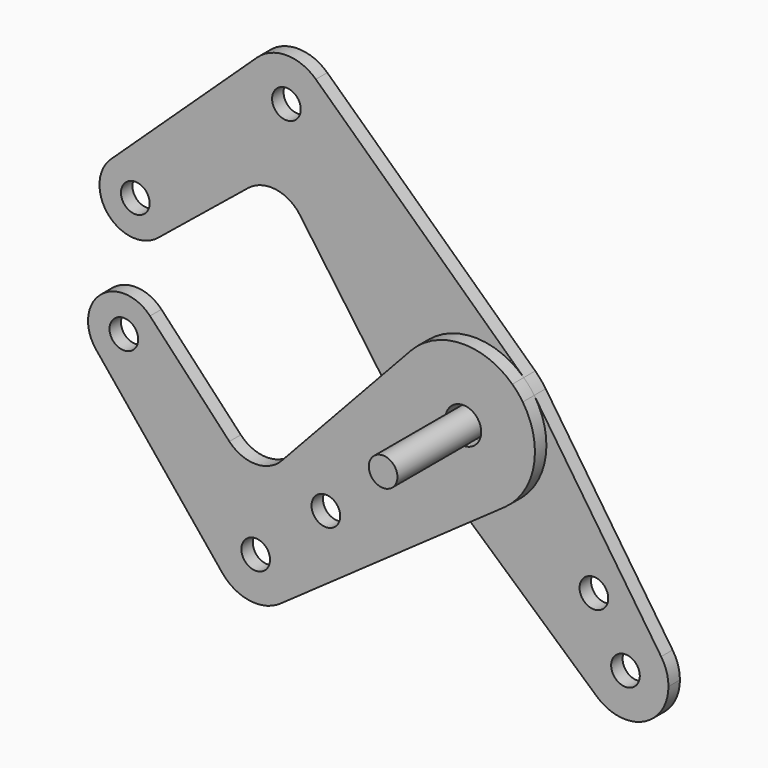
from build123d import *

# Parameters (mm, degrees)
F0_R     = 3.175
F0_R_2   = 3.96875
F1_DEPTH = 3.175
F2_DEPTH = 3.175
F3_DEPTH = 25.4


# Not quite as in the source:
# - a feature names something its author has since deleted; it is built from what else it names


with BuildPart() as f1:
    # F0 (on Front) → F1 (new body)
    with BuildSketch(Plane.XZ):
        with BuildLine():
            ThreePointArc((21.168407994, 17.4724150988), (32.2496948497, 22.5266363925), (43.6506851161, 18.2420719796))
            Line((43.6506851161, 18.2420719796), (-2.4416753004, 61.4557481855))
            ThreePointArc((-2.4416753004, 61.4557481855), (-0.2162960867, 58.2934233078), (0.5686178911, 54.5070634035))
            ThreePointArc((0.5686178911, 54.5070634035), (-12.7427420132, 45.7669773813), (-15.4710889174, 61.4557481855))
            Line((-15.4710889174, 61.4557481855), (-47.8775973584, 31.0731782742))
            ThreePointArc((-47.8775973584, 31.0731782742), (-39.2933750978, 32.5660126411), (-34.511175018, 25.2826076226))
            ThreePointArc((-34.511175018, 25.2826076226), (-35.2826057932, 21.8691990453), (-37.4469502912, 19.1192760553))
            Line((-37.4469502912, 19.1192760553), (-17.4168982381, 35.3742520435))
            ThreePointArc((-17.4168982381, 35.3742520435), (-11.3398687202, 37.0752466303), (-5.9425206073, 33.8053378098))
            Line((-5.9425206073, 33.8053378098), (12.3676167081, 8.0098658563))
            Line((12.3676167081, 8.0098658563), (21.168407994, 17.4724150988))
        make_face()
        with BuildLine():
            ThreePointArc((0.5686178911, 54.5070634035), (-0.2162960867, 58.2934233078), (-2.4416753004, 61.4557481855))
            ThreePointArc((-2.4416753004, 61.4557481855), (-8.9563821089, 64.0320634035), (-15.4710889174, 61.4557481855))
            ThreePointArc((-15.4710889174, 61.4557481855), (-12.7427420132, 45.7669773813), (0.5686178911, 54.5070634035))
        make_face()
        with Locations((-8.9563821089, 54.5070634035)):
            Circle(F0_R, mode=Mode.SUBTRACT)
        with BuildLine():
            ThreePointArc((-34.511175018, 25.2826076226), (-39.2933750978, 32.5660126411), (-47.8775973584, 31.0731782742))
            ThreePointArc((-47.8775973584, 31.0731782742), (-48.4294416089, 20.0639548045), (-37.4469502912, 19.1192760553))
            ThreePointArc((-37.4469502912, 19.1192760553), (-35.2826057932, 21.8691990453), (-34.511175018, 25.2826076226))
        make_face()
        with Locations((-42.448675018, 25.2826076226)):
            Circle(F0_R, mode=Mode.SUBTRACT)
        with BuildLine():
            ThreePointArc((48.6678404353, 6.6609306763), (47.9771603326, 11.292566916), (45.9652194266, 15.52118218))
            ThreePointArc((45.9652194266, 15.52118218), (44.8847270854, 16.9469358407), (43.6506851161, 18.2420719796))
            ThreePointArc((43.6506851161, 18.2420719796), (32.2496948497, 22.5266363925), (21.168407994, 17.4724150988))
            ThreePointArc((21.168407994, 17.4724150988), (16.9523480083, 7.7070782137), (19.8475346273, -2.5279039906))
            ThreePointArc((19.8475346273, -2.5279039906), (20.9635537477, -3.926023629), (22.229787853, -5.1897041229))
            ThreePointArc((22.229787853, -5.1897041229), (31.8827140076, -9.1879587134), (41.9298775136, -6.3209866871))
            ThreePointArc((41.9298775136, -6.3209866871), (46.8830158887, -0.6522478865), (48.6678404353, 6.6609306763))
        make_face()
        with Locations((32.7928404353, 6.6609306763)):
            Circle(F0_R_2, mode=Mode.SUBTRACT)
        with BuildLine():
            ThreePointArc((59.8543869213, -38.726356385), (59.9298350891, -24.4390555964), (74.0956458655, -26.2998246032))
            Line((74.0956458655, -26.2998246032), (45.9652194266, 15.52118218))
            ThreePointArc((45.9652194266, 15.52118218), (47.9771603326, 11.292566916), (48.6678404353, 6.6609306763))
            ThreePointArc((48.6678404353, 6.6609306763), (46.8830158887, -0.6522478865), (41.9298775136, -6.3209866871))
            Line((41.9298775136, -6.3209866871), (31.63109975, -13.5695549573))
            Line((31.63109975, -13.5695549573), (59.8543869213, -38.726356385))
        make_face()
        with Locations((59.1909500346, -18.7631345147)):
            Circle(F0_R, mode=Mode.SUBTRACT)
        with BuildLine():
            Line((22.229787853, -5.1897041229), (31.63109975, -13.5695549573))
            Line((31.63109975, -13.5695549573), (41.9298775136, -6.3209866871))
            ThreePointArc((41.9298775136, -6.3209866871), (31.8827140076, -9.1879587134), (22.229787853, -5.1897041229))
        make_face()
        with BuildLine():
            ThreePointArc((19.8475346273, -2.5279039906), (16.9523480083, 7.7070782137), (21.168407994, 17.4724150988))
            Line((21.168407994, 17.4724150988), (12.3676167081, 8.0098658563))
            Line((12.3676167081, 8.0098658563), (19.8475346273, -2.5279039906))
        make_face()
        with BuildLine():
            ThreePointArc((59.8543869213, -38.726356385), (70.088227935, -40.3077379996), (75.7172184707, -31.6159755055))
            ThreePointArc((75.7172184707, -31.6159755055), (75.3028104091, -28.8369937617), (74.0956458655, -26.2998246032))
            ThreePointArc((74.0956458655, -26.2998246032), (59.9298350891, -24.4390555964), (59.8543869213, -38.726356385))
        make_face()
        with Locations((66.1922184707, -31.6159755055)):
            Circle(F0_R, mode=Mode.SUBTRACT)
    extrude(amount=-F1_DEPTH)


with BuildPart() as f2:
    # F0 (on Front) → F2 (new body)
    with BuildSketch(Plane.XZ):
        with Locations((32.7928404353, 6.6609306763)):
            Circle(F0_R)
    extrude(amount=F2_DEPTH)

    # F0 (on Front) → F3 (join)
    with BuildSketch(Plane.XZ):
        with Locations((32.7928404353, 6.6609306763)):
            Circle(F0_R)
    extrude(amount=F3_DEPTH)


with BuildPart() as f2b:
    # F0 (on Front) → F2, piece 2 (new body)
    with BuildSketch(Plane.XZ):
        with BuildLine():
            ThreePointArc((48.6678404353, 6.6609306763), (47.9771603326, 11.292566916), (45.9652194266, 15.52118218))
            ThreePointArc((45.9652194266, 15.52118218), (44.8847270854, 16.9469358407), (43.6506851161, 18.2420719796))
            ThreePointArc((43.6506851161, 18.2420719796), (32.2496948497, 22.5266363925), (21.168407994, 17.4724150988))
            ThreePointArc((21.168407994, 17.4724150988), (16.9523480083, 7.7070782137), (19.8475346273, -2.5279039906))
            ThreePointArc((19.8475346273, -2.5279039906), (20.9635537477, -3.926023629), (22.229787853, -5.1897041229))
            ThreePointArc((22.229787853, -5.1897041229), (31.8827140076, -9.1879587134), (41.9298775136, -6.3209866871))
            ThreePointArc((41.9298775136, -6.3209866871), (46.8830158887, -0.6522478865), (48.6678404353, 6.6609306763))
        make_face()
        with Locations((32.7928404353, 6.6609306763)):
            Circle(F0_R_2, mode=Mode.SUBTRACT)
        with BuildLine():
            Line((-7.7419969901, -41.2814433271), (31.63109975, -13.5695549573))
            Line((31.63109975, -13.5695549573), (22.229787853, -5.1897041229))
            ThreePointArc((22.229787853, -5.1897041229), (20.9635537477, -3.926023629), (19.8475346273, -2.5279039906))
            Line((19.8475346273, -2.5279039906), (12.3676167081, 8.0098658563))
            Line((12.3676167081, 8.0098658563), (-7.4631189723, -13.3120024615))
            ThreePointArc((-7.4631189723, -13.3120024615), (-13.2594776313, -15.8437444101), (-19.0659058445, -13.3351825907))
            Line((-19.0659058445, -13.3351825907), (-36.6581043663, 5.4289223404))
            ThreePointArc((-36.6581043663, 5.4289223404), (-35.067395969, 2.9190111085), (-34.511175018, 0))
            ThreePointArc((-34.511175018, 0), (-39.7951432267, -7.4808204953), (-48.6120065852, -5.0017247268))
            Line((-48.6120065852, -5.0017247268), (-20.6202171177, -39.4943625812))
            ThreePointArc((-20.6202171177, -39.4943625812), (-20.0372197924, -26.8358187348), (-7.3956423811, -25.9588131796))
            ThreePointArc((-7.3956423811, -25.9588131796), (-4.6731134737, -29.2965551642), (-3.699219237, -33.4922929091))
            ThreePointArc((-3.699219237, -33.4922929091), (-4.3961637904, -37.0687523357), (-6.3850065401, -40.1218324621))
            ThreePointArc((-6.3850065401, -40.1218324621), (-7.0362782136, -40.7334952188), (-7.7419969901, -41.2814433271))
        make_face()
        with Locations((2.3257738993, -19.9237955822)):
            Circle(F0_R, mode=Mode.SUBTRACT)
        with BuildLine():
            Line((22.229787853, -5.1897041229), (31.63109975, -13.5695549573))
            Line((31.63109975, -13.5695549573), (41.9298775136, -6.3209866871))
            ThreePointArc((41.9298775136, -6.3209866871), (31.8827140076, -9.1879587134), (22.229787853, -5.1897041229))
        make_face()
        with BuildLine():
            ThreePointArc((-20.6202171177, -39.4943625812), (-14.533436061, -42.9268875643), (-7.7419969901, -41.2814433271))
            ThreePointArc((-7.7419969901, -41.2814433271), (-7.0362782136, -40.7334952188), (-6.3850065401, -40.1218324621))
            Line((-6.3850065401, -40.1218324621), (-6.8903244606, -33.0403228209))
            Line((-6.8903244606, -33.0403228209), (-7.3956423811, -25.9588131796))
            ThreePointArc((-7.3956423811, -25.9588131796), (-20.0372197924, -26.8358187348), (-20.6202171177, -39.4943625812))
        make_face()
        with BuildLine():
            ThreePointArc((-10.049219237, -33.4922929091), (-16.3972054455, -33.6053571438), (-10.0572718488, -33.266307865))
            ThreePointArc((-10.0572718488, -33.266307865), (-10.0512330286, -33.3792286743), (-10.049219237, -33.4922929091))
        make_face(mode=Mode.SUBTRACT)
        with BuildLine():
            ThreePointArc((19.8475346273, -2.5279039906), (16.9523480083, 7.7070782137), (21.168407994, 17.4724150988))
            Line((21.168407994, 17.4724150988), (12.3676167081, 8.0098658563))
            Line((12.3676167081, 8.0098658563), (19.8475346273, -2.5279039906))
        make_face()
        with BuildLine():
            Line((-6.8903244606, -33.0403228209), (-6.3850065401, -40.1218324621))
            ThreePointArc((-6.3850065401, -40.1218324621), (-4.3961637904, -37.0687523357), (-3.699219237, -33.4922929091))
            ThreePointArc((-3.699219237, -33.4922929091), (-4.6731134737, -29.2965551642), (-7.3956423811, -25.9588131796))
            Line((-7.3956423811, -25.9588131796), (-6.8903244606, -33.0403228209))
        make_face()
        with BuildLine():
            ThreePointArc((-36.6581043663, 5.4289223404), (-47.667327836, 5.9807665909), (-48.6120065852, -5.0017247268))
            ThreePointArc((-48.6120065852, -5.0017247268), (-39.7951432267, -7.4808204953), (-34.511175018, 0))
            ThreePointArc((-34.511175018, 0), (-35.067395969, 2.9190111085), (-36.6581043663, 5.4289223404))
        make_face()
        with Locations((-42.448675018, 0)):
            Circle(F0_R, mode=Mode.SUBTRACT)
    extrude(amount=F2_DEPTH)


solid = Compound([f1.part, f2.part, f2b.part])
